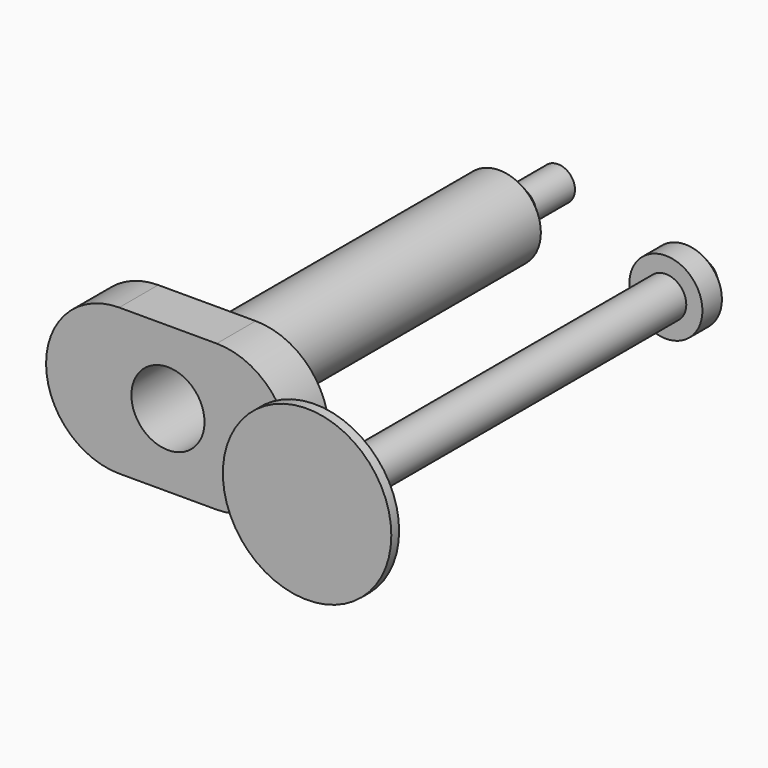
from build123d import *

# Parameters (mm, degrees)
F0_R      = 10.795
F1_DEPTH  = 101.6
F2_SIZE   = 6.35
F3_DEPTH  = 12.7
F4_W      = 63.5
F4_H      = 38.1
F5_DEPTH  = 12.7
F6_R      = 19.04999
F7_R      = 9.525
F8_DEPTH  = 109.06528
F9_R      = 2.3789918441
F10_DEPTH = 87.48307
F11_DEPTH = 12.7
F0_R_2    = 9.525
F12_DEPTH = 12.7
F13_SIZE  = 6.35
F14_R     = 5.3195531206
F15_DEPTH = 114.3
F16_R     = 21.9454627566
F17_DEPTH = 2.54


# Not quite as in the source:
# - a fillet or chamfer is up to 0.001 mm smaller than in the source, because OpenCascade refuses the exact size


with BuildPart() as f1:
    # F0 (on Front) → F1 (new body)
    with BuildSketch(Plane.XZ):
        Circle(F0_R)
    extrude(amount=F1_DEPTH)

    # F2
    f2_edges = [f1.edges().sort_by_distance(p)[0] for p in [
        (-10.795, 0, 0),
    ]]
    chamfer(f2_edges, length=F2_SIZE)

    # F3 (add): a face of the model
    f3_faces = [f1.faces().sort_by_distance(p)[0] for p in [
        (0, 0, 0),
    ]]
    extrude(f3_faces, amount=F3_DEPTH)

    # F4 (on face) → F5 (join)
    with BuildSketch(Plane.XZ.offset(101.6)):
        Rectangle(F4_W, F4_H)
    extrude(amount=F5_DEPTH)

    # F6 (radius 19.05 in the source; OpenCascade refuses exactly that, so slightly less here)
    f6_edges = [f1.edges().sort_by_distance(p)[0] for p in [
        (-31.75, -107.95, 19.05),
        (31.75, -107.95, 19.05),
        (31.75, -107.95, -19.05),
        (-31.75, -107.95, -19.05),
    ]]
    fillet(f6_edges, radius=F6_R)

    # F7 (on face) → F8 (cut)
    with BuildSketch(Plane.XZ.offset(114.3)):
        Circle(F7_R)
    extrude(amount=-F8_DEPTH, mode=Mode.SUBTRACT)

    # F9 (on face) → F10 (cut)
    with BuildSketch(Plane(origin=(0, 12.7, 0), x_dir=(-1, 0, 0), z_dir=(0, 1, 0))):
        Circle(F9_R)
    extrude(amount=-F10_DEPTH, mode=Mode.SUBTRACT)


with BuildPart() as f11:
    # F0 (on Front) → F11 (new body)
    with BuildSketch(Plane.XZ):
        Circle(F0_R)
    extrude(amount=F11_DEPTH)


with BuildPart() as f12:
    # F0 (on Front) → F12 (new body)
    with BuildSketch(Plane.XZ):
        with Locations((48.4419576824, 0)):
            Circle(F0_R_2)
    extrude(amount=F12_DEPTH)

    # F13
    f13_edges = [f12.edges().sort_by_distance(p)[0] for p in [
        (38.916958, 0, 0),
    ]]
    chamfer(f13_edges, length=F13_SIZE)

    # F14 (on face) → F15 (join)
    with BuildSketch(Plane.XZ.offset(12.7)):
        with Locations((48.4419576824, 0)):
            Circle(F14_R)
    extrude(amount=F15_DEPTH)

    # F16 (on face) → F17 (join)
    with BuildSketch(Plane.XZ.offset(127)):
        with Locations((48.4419576824, 0)):
            Circle(F16_R)
    extrude(amount=F17_DEPTH)


solid = Compound([f1.part, f12.part])
